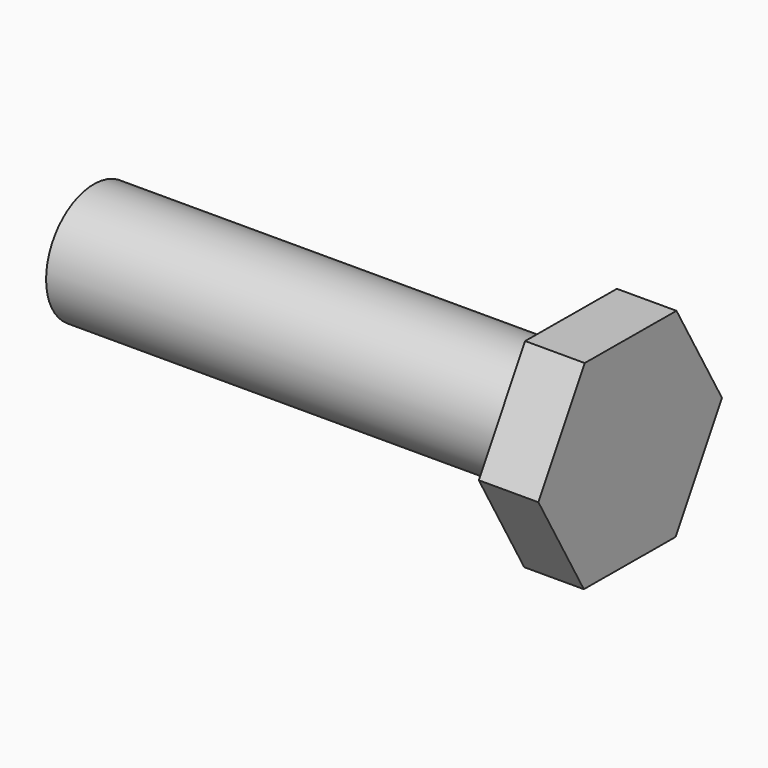
from build123d import *

# Parameters (mm, degrees)
F1_DEPTH = 3
F2_R     = 3
F3_DEPTH = 24


# Not quite as in the source:
# - a feature names something its author has since deleted; it is built from what else it names


with BuildPart() as f1:
    # F0 (on Right) → F1 (new body)
    with BuildSketch(Plane.YZ):
        Polygon((5.7734155665, -0.0317179771), (2.9141763572, 4.9840655586), (-2.8592392093, 5.0157835357), (-5.7734155665, 0.0317179771), (-2.9141763572, -4.9840655586), (2.8592392093, -5.0157835357), align=None)
    extrude(amount=F1_DEPTH)

    # F2 (on face) → F3 (join)
    with BuildSketch(Plane(origin=(0, 0, 0), x_dir=(0, -1, 0), z_dir=(-1, 0, 0))):
        Circle(F2_R)
    extrude(amount=F3_DEPTH)


solid = f1.part
